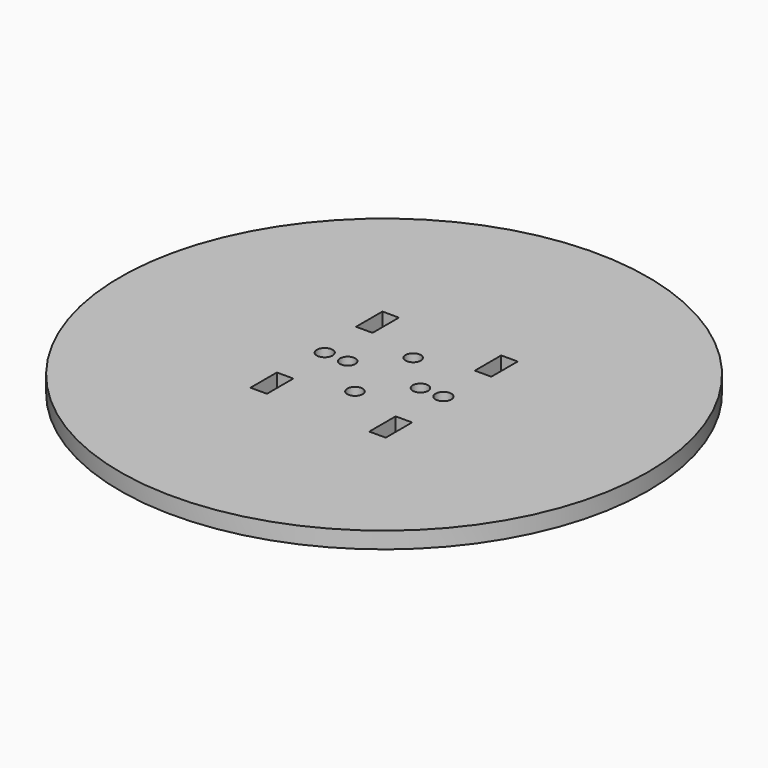
from build123d import *

# Parameters (mm, degrees)
F0_R     = 50.8
F0_W     = 3.175
F0_H     = 6.35
F0_R_2   = 1.4732
F0_R_3   = 1.524
F1_DEPTH = 3.175


# Not quite as in the source:
# - a length typed as a fraction of an inch, garbled in the dataset ("3 / 203.2 mm" for 3/8 in), is restored


with BuildPart() as f1:
    # F0 (on Top) → F1 (new body)
    with BuildSketch(Plane.XY):
        Circle(F0_R)
        with Locations((-11.43, -12.7)):
            Rectangle(F0_W, F0_H, mode=Mode.SUBTRACT)
        with Locations((0, -7)):
            Circle(F0_R_2, mode=Mode.SUBTRACT)
        with Locations((-11.43, 0)):
            Circle(F0_R_3, mode=Mode.SUBTRACT)
        with Locations((-7, 0)):
            Circle(F0_R_2, mode=Mode.SUBTRACT)
        with Locations((11.43, -12.7)):
            Rectangle(F0_W, F0_H, mode=Mode.SUBTRACT)
        with Locations((7, 0)):
            Circle(F0_R_2, mode=Mode.SUBTRACT)
        with Locations((11.43, 0)):
            Circle(F0_R_3, mode=Mode.SUBTRACT)
        with Locations((0, 7)):
            Circle(F0_R_2, mode=Mode.SUBTRACT)
        with Locations((-11.43, 12.7)):
            Rectangle(F0_W, F0_H, mode=Mode.SUBTRACT)
        with Locations((11.43, 12.7)):
            Rectangle(F0_W, F0_H, mode=Mode.SUBTRACT)
    extrude(amount=F1_DEPTH)


solid = f1.part
